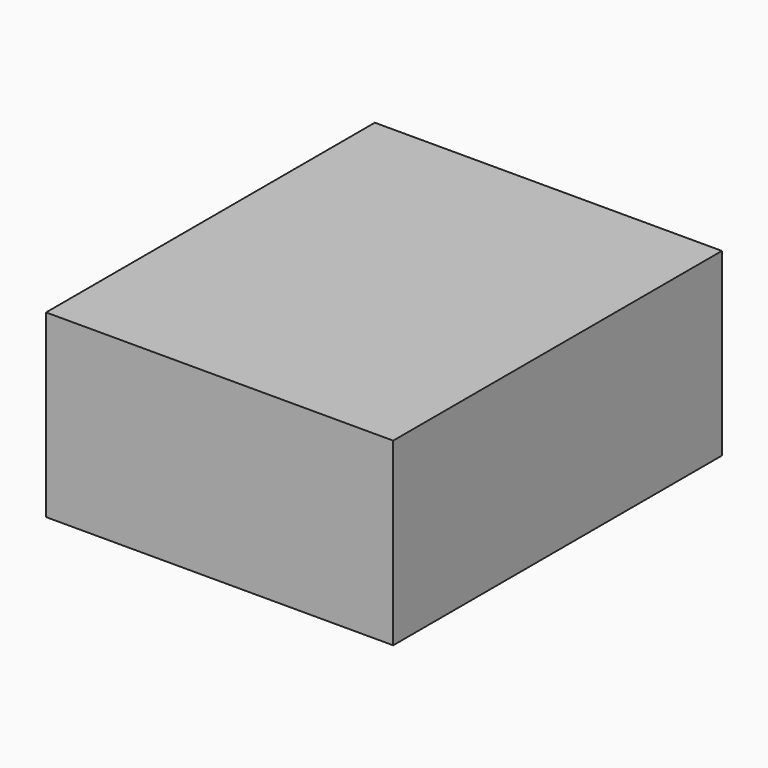
from build123d import *

# Parameters (mm, degrees)
F1_DEPTH  = 63.5
F0_W      = 25.4
F0_H      = 19.05
F2_DEPTH  = 25.4
F3_DEPTH  = 7.9375
F5_R      = 5.08
F9_W      = 48.9222034812
F9_H      = 57.9138733447
F12_DEPTH = 25.4


# Not quite as in the source:
# - the program builds the solid bodies; features that only make, move or delete a surface that nothing else refers to are left out


with BuildPart() as f1:
    # F0 (on Front) → F1 (new body, symmetric)
    with BuildSketch(Plane.XZ):
        Polygon((22.225, 9.525), (-41.275, 9.525), (-41.275, -9.525), (41.275, -9.525), (41.275, 9.525), align=None)
    extrude(amount=F1_DEPTH, both=True)

    # F0 (on Front) → F2 (join, symmetric)
    with BuildSketch(Plane.XZ):
        with BuildLine():
            Line((22.225, 27.0002), (22.225, 9.525))
            Line((22.225, 9.525), (41.275, 9.525))
            Line((41.275, 9.525), (41.275, 27.0002))
            ThreePointArc((41.275, 27.0002), (45.9246798487, 38.2255201513), (57.15, 42.8752))
            Line((57.15, 42.8752), (60.325, 42.8752))
            Line((60.325, 42.8752), (60.325, 61.9252))
            Line((60.325, 61.9252), (57.15, 61.9252))
            add(Edge.make_bspline(
                [(53.8854342407, 61.7722898912), (54.9842067368, 61.8365871986), (56.0728453275, 61.8876096574), (57.15, 61.9252)],
                knots=[108.5245810491, 108.5245810491, 108.5245810491, 108.5245810491, 111.5045361635, 111.5045361635, 111.5045361635, 111.5045361635], degree=3))
            ThreePointArc((53.8854342407, 61.7722898912), (31.3258777096, 50.5133948686), (22.225, 27.0002))
        make_face()
        with Locations((73.025, 52.4002)):
            Rectangle(F0_W, F0_H)
    extrude(amount=F2_DEPTH, both=True)

    # F0 (on Front) → F3 (join, symmetric)
    with BuildSketch(Plane.XZ):
        with BuildLine():
            add(Edge.make_bspline(
                [(-41.275, 9.525), (-39.5856284224, 39.4828766469), (13.870125209, 59.4306981306), (53.8854342407, 61.7722898912)],
                knots=[0, 0, 0, 0, 108.5245810491, 108.5245810491, 108.5245810491, 108.5245810491], degree=3))
            Line((-41.275, 9.525), (22.225, 9.525))
            Line((22.225, 9.525), (22.225, 27.0002))
            ThreePointArc((22.225, 27.0002), (31.3258777096, 50.5133948686), (53.8854342407, 61.7722898912))
        make_face()
    extrude(amount=F3_DEPTH, both=True)

    # F0 (on Front) → F4 (revolve)
    with BuildSketch(Plane.XZ):
        Polygon((85.725, 66.675), (85.725, 61.9252), (85.725, 42.8752), (85.725, 38.1), (111.125, 38.1), (111.125, 66.675), align=None)
    revolve(axis=Axis((85.725, 0, 52.3875), (0, 0, 1)))

    # F5
    f5_edges = [f1.edges().sort_by_distance(p)[0] for p in [
        (41.275, -63.5, 0),
        (-41.275, -63.5, 0),
        (41.275, 63.5, 0),
        (-41.275, 63.5, 0),
    ]]
    fillet(f5_edges, radius=F5_R)


with BuildPart() as f12:
    # F9 (on face) → F12 (new body)
    with BuildSketch(Plane.XY.offset(66.675)):
        with Locations((130.5457092822, -90.9018423408)):
            Rectangle(F9_W, F9_H)
    extrude(amount=F12_DEPTH)


solid = f12.part
